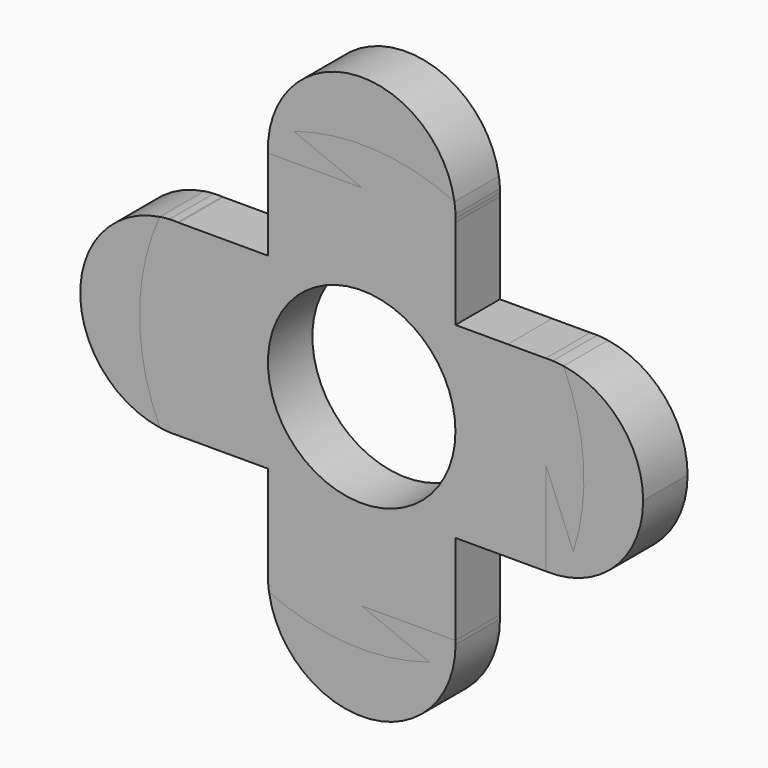
from build123d import *
from build123d import SkipClean  # not in build123d's __all__

# Parameters (mm, degrees)
F0_R     = 25.4
F1_DEPTH = 6.35
F2_R     = 10.715625
F3_DEPTH = 6.351
F5_DEPTH = 6.351
F7_DEPTH = 6.35


# Not quite as in the source:
# - ends of sketch curves that miss each other by under 0.0002 mm in the source are joined


with BuildPart() as f1:
    # F0 (on Front) → F1 (new body)
    with BuildSketch(Plane.XZ):
        Circle(F0_R)
    extrude(amount=F1_DEPTH)

    # F2 (on face) → F3 (cut, through all)
    with BuildSketch(Plane.XZ.offset(6.35)):
        Circle(F2_R)
    extrude(amount=-F3_DEPTH, mode=Mode.SUBTRACT)

    # F4 (on face) → F5 (cut, through all)
    with BuildSketch(Plane.XZ.offset(6.35)):
        Polygon((-16.6851454689, 10.715625), (-10.715625, 10.715625), (-10.715625, 16.6851454689), (-14.959796627, 14.959796627), align=None)
        with BuildLine():
            Line((-14.959796627, 14.959796627), (-10.715625, 16.6851454689))
            Line((-10.715625, 16.6851454689), (-10.715625, 21.0412820273))
            ThreePointArc((-10.715625, 21.0412820273), (-10.7231093189, 21.441908849), (-10.715625, 21.8425356707))
            Line((-10.715625, 21.8425356707), (-10.715625, 23.0290117213))
            ThreePointArc((-10.715625, 23.0290117213), (-11.3239040523, 22.7360769926), (-11.9241826151, 22.4270789217))
            Line((-11.9241826151, 22.4270789217), (-14.959796627, 14.959796627))
        make_face()
        with BuildLine():
            Line((-20.9014356742, 10.715625), (-16.6851454689, 10.715625))
            Line((-16.6851454689, 10.715625), (-14.959796627, 14.959796627))
            Line((-14.959796627, 14.959796627), (-22.4270789217, 11.9241826151))
            ThreePointArc((-22.4270789217, 11.9241826151), (-22.7360769926, 11.3239040523), (-23.0290117213, 10.715625))
            Line((-23.0290117213, 10.715625), (-21.9888344018, 10.715625))
            ThreePointArc((-21.9888344018, 10.715625), (-21.517375938, 10.7291661682), (-21.0457778798, 10.7219746652))
            ThreePointArc((-21.0457778798, 10.7219746652), (-20.9735960889, 10.7190427964), (-20.9014356742, 10.715625))
        make_face()
        Polygon((-10.715625, -16.6889140547), (-10.715625, -10.7183040998), (-16.6844990564, -10.7197962397), (-14.9584916016, -14.9648416016), align=None)
        Polygon((10.721975, 16.6873822364), (10.721975, 10.7183053524), (16.6882676196, 10.7197968469), (14.9635371125, 14.9635367777), align=None)
        with BuildLine():
            ThreePointArc((-10.715625, 21.8425356707), (-10.7231093189, 21.441908849), (-10.715625, 21.0412820273))
            Line((-10.715625, 21.0412820273), (-10.715625, 21.8425356707))
        make_face()
        with BuildLine():
            Line((-10.715625, 21.8425356707), (-10.715625, 21.0412820273))
            Line((-10.715625, 21.0412820273), (0, 21.0412820273))
            Line((0, 21.0412820273), (0.0045507281, 21.0431319981))
            Line((0.0045507281, 21.0431319981), (-7.7418402479, 24.1914015629))
            ThreePointArc((-7.7418402479, 24.1914015629), (-9.1859591102, 23.6807549547), (-10.596671596, 23.0839890635))
            ThreePointArc((-10.596671596, 23.0839890635), (-10.6742064582, 22.4649926613), (-10.715625, 21.8425356707))
        make_face()
        with BuildLine():
            Line((-22.4270789217, 11.9241826151), (-14.959796627, 14.959796627))
            Line((-14.959796627, 14.959796627), (-11.9241826151, 22.4270789217))
            ThreePointArc((-11.9241826151, 22.4270789217), (-17.9605122421, 17.9605122421), (-22.4270789217, 11.9241826151))
        make_face()
        with BuildLine():
            Line((-10.715625, -21.0430976268), (-10.715625, -16.6889140547))
            Line((-10.715625, -16.6889140547), (-14.9584916016, -14.9648416016))
            Line((-14.9584916016, -14.9648416016), (-11.9244537164, -22.4269347787))
            ThreePointArc((-11.9244537164, -22.4269347787), (-11.3240414708, -22.7360085496), (-10.715625, -23.0290117213))
            Line((-10.715625, -23.0290117213), (-10.715625, -21.8405802232))
            ThreePointArc((-10.715625, -21.8405802232), (-10.7230390601, -21.441838925), (-10.715625, -21.0430976268))
        make_face()
        with BuildLine():
            Line((-14.9584916016, -14.9648416016), (-16.6844990564, -10.7197962397))
            Line((-16.6844990564, -10.7197962397), (-21.0123347342, -10.7208781415))
            ThreePointArc((-21.0123347342, -10.7208781415), (-21.0263755955, -10.7214357653), (-21.0404171751, -10.721975))
            ThreePointArc((-21.0404171751, -10.721975), (-21.4565047306, -10.7296046859), (-21.8725751819, -10.7210931903))
            Line((-21.8725751819, -10.7210931903), (-23.0263322368, -10.7213816143))
            ThreePointArc((-23.0263322368, -10.7213816143), (-22.7327836194, -11.3305140622), (-22.4231246927, -11.9316167813))
            Line((-22.4231246927, -11.9316167813), (-14.9584916016, -14.9648416016))
        make_face()
        Polygon((16.6889139739, -10.7156253348), (10.721975, -10.7156253348), (10.721975, -16.6836133856), (14.9648415328, -14.9584918676), align=None)
        with BuildLine():
            Line((10.721975, 21.0412820273), (10.721975, 16.6873822364))
            Line((10.721975, 16.6873822364), (14.9635371125, 14.9635367777))
            Line((14.9635371125, 14.9635367777), (11.9318881389, 22.4229802979))
            ThreePointArc((11.9318881389, 22.4229802979), (11.3309445253, 22.7325690621), (10.721975, 23.0260559389))
            Line((10.721975, 23.0260559389), (10.721975, 21.8425356707))
            ThreePointArc((10.721975, 21.8425356707), (10.727588076, 21.6422572114), (10.7294593189, 21.441908849))
            ThreePointArc((10.7294593189, 21.441908849), (10.727588076, 21.2415604866), (10.721975, 21.0412820273))
        make_face()
        with BuildLine():
            Line((14.9635371125, 14.9635367777), (16.6882676196, 10.7197968469))
            Line((16.6882676196, 10.7197968469), (21.0404868941, 10.7208848444))
            ThreePointArc((21.0404868941, 10.7208848444), (21.4451864116, 10.7286236807), (21.8498897476, 10.7210871844))
            Line((21.8498897476, 10.7210871844), (23.0263323927, 10.7213812796))
            ThreePointArc((23.0263323927, 10.7213812796), (22.7327152374, 11.3306512582), (22.4229804989, 11.9318877612))
            Line((22.4229804989, 11.9318877612), (14.9635371125, 14.9635367777))
        make_face()
        with BuildLine():
            Line((-10.715625, 23.0290117213), (-10.715625, 21.8425356707))
            ThreePointArc((-10.715625, 21.8425356707), (-10.6742064582, 22.4649926613), (-10.596671596, 23.0839890635))
            ThreePointArc((-10.596671596, 23.0839890635), (-10.6561837529, 23.0565771055), (-10.715625, 23.0290117213))
        make_face()
        with BuildLine():
            Line((-11.9244537164, -22.4269347787), (-14.9584916016, -14.9648416016))
            Line((-14.9584916016, -14.9648416016), (-22.4231246927, -11.9316167813))
            ThreePointArc((-22.4231246927, -11.9316167813), (-17.9576435149, -17.9633805112), (-11.9244537164, -22.4269347787))
        make_face()
        with BuildLine():
            Line((14.9648415328, -14.9584918676), (10.721975, -16.6836133856))
            Line((10.721975, -16.6836133856), (10.721975, -21.0430976268))
            ThreePointArc((10.721975, -21.0430976268), (10.7275353849, -21.2424338153), (10.7293890601, -21.441838925))
            ThreePointArc((10.7293890601, -21.441838925), (10.7275353849, -21.6412440348), (10.721975, -21.8405802232))
            Line((10.721975, -21.8405802232), (10.721975, -23.0260559389))
            ThreePointArc((10.721975, -23.0260559389), (11.3308069807, -22.7326376201), (11.9316167956, -22.4231246851))
            Line((11.9316167956, -22.4231246851), (14.9648415328, -14.9584918676))
        make_face()
        with BuildLine():
            Line((21.0458457391, -10.7156253348), (16.6889139739, -10.7156253348))
            Line((16.6889139739, -10.7156253348), (14.9648415328, -14.9584918676))
            Line((14.9648415328, -14.9584918676), (22.4269345702, -11.9244541084))
            ThreePointArc((22.4269345702, -11.9244541084), (22.7360083683, -11.3240418348), (23.0290115655, -10.7156253348))
            Line((23.0290115655, -10.7156253348), (21.8498897476, -10.7156253348))
            ThreePointArc((21.8498897476, -10.7156253348), (21.4478677434, -10.7231621662), (21.0458457391, -10.7156253348))
        make_face()
        with BuildLine():
            Line((10.721975, -21.0430976268), (0, -21.0430976268))
            Line((0, -21.0430976268), (7.7450996927, -24.1903582187))
            ThreePointArc((7.7450996927, -24.1903582187), (9.1910155426, -23.678792902), (10.6034192636, -23.0808903624))
            ThreePointArc((10.6034192636, -23.0808903624), (10.6807217402, -22.462458185), (10.721975, -21.8405802232))
            Line((10.721975, -21.8405802232), (10.721975, -21.0430976268))
        make_face()
        with BuildLine():
            ThreePointArc((10.7293890601, -21.441838925), (10.7275353849, -21.2424338153), (10.721975, -21.0430976268))
            Line((10.721975, -21.0430976268), (10.721975, -21.8405802232))
            ThreePointArc((10.721975, -21.8405802232), (10.7275353849, -21.6412440348), (10.7293890601, -21.441838925))
        make_face()
        with BuildLine():
            ThreePointArc((-23.0806092952, 10.6040310525), (-22.536149575, 10.6737961307), (-21.9888344018, 10.715625))
            Line((-21.9888344018, 10.715625), (-23.0290117213, 10.715625))
            ThreePointArc((-23.0290117213, 10.715625), (-23.0548780277, 10.6598592451), (-23.0806092952, 10.6040310525))
        make_face()
        with BuildLine():
            Line((11.9318881389, 22.4229802979), (14.9635371125, 14.9635367777))
            Line((14.9635371125, 14.9635367777), (22.4229804989, 11.9318877612))
            ThreePointArc((22.4229804989, 11.9318877612), (17.9605123934, 17.9605120909), (11.9318881389, 22.4229802979))
        make_face()
        with BuildLine():
            ThreePointArc((10.6035074316, 23.0808498576), (10.6807078337, 22.4634116022), (10.721975, 21.8425356707))
            Line((10.721975, 21.8425356707), (10.721975, 23.0260559389))
            ThreePointArc((10.721975, 23.0260559389), (10.6627764128, 23.053528996), (10.6035074316, 23.0808498576))
        make_face()
        with BuildLine():
            ThreePointArc((-10.5965833938, -23.0840295525), (-10.674220495, -22.4640392514), (-10.715625, -21.8405802232))
            Line((-10.715625, -21.8405802232), (-10.715625, -23.0290117213))
            ThreePointArc((-10.715625, -23.0290117213), (-10.6561397042, -23.0565974637), (-10.5965833938, -23.0840295525))
        make_face()
        with BuildLine():
            Line((-23.0263322368, -10.7213816143), (-21.8725751819, -10.7210931903))
            ThreePointArc((-21.8725751819, -10.7210931903), (-22.4781957728, -10.6797622384), (-23.0805097356, -10.60424775))
            ThreePointArc((-23.0805097356, -10.60424775), (-23.0534953804, -10.6628490914), (-23.0263322368, -10.7213816143))
        make_face()
        with BuildLine():
            Line((22.4269345702, -11.9244541084), (14.9648415328, -14.9584918676))
            Line((14.9648415328, -14.9584918676), (11.9316167956, -22.4231246851))
            ThreePointArc((11.9316167956, -22.4231246851), (17.96338036, -17.9576436662), (22.4269345702, -11.9244541084))
        make_face()
        with BuildLine():
            Line((21.043166974, 0), (21.0458457391, -10.7156253348))
            Line((21.0458457391, -10.7156253348), (21.8498897476, -10.7156253348))
            ThreePointArc((21.8498897476, -10.7156253348), (22.4684041732, -10.6745013006), (23.083509992, -10.5977151524))
            ThreePointArc((23.083509992, -10.5977151524), (23.6805472866, -9.1864944461), (24.19140152, -7.7418403819))
            Line((24.19140152, -7.7418403819), (21.0440741561, 0.0022325353))
            Line((21.0440741561, 0.0022325353), (21.043166974, 0))
        make_face()
        with BuildLine():
            Line((21.8498897476, -10.7156253348), (21.0458457391, -10.7156253348))
            ThreePointArc((21.0458457391, -10.7156253348), (21.4478677434, -10.7231621662), (21.8498897476, -10.7156253348))
        make_face()
        with BuildLine():
            Line((10.721975, -23.0260559389), (10.721975, -21.8405802232))
            ThreePointArc((10.721975, -21.8405802232), (10.6807217402, -22.462458185), (10.6034192636, -23.0808903624))
            ThreePointArc((10.6034192636, -23.0808903624), (10.662732381, -23.0535493617), (10.721975, -23.0260559389))
        make_face()
        with BuildLine():
            Line((23.0263323927, 10.7213812796), (21.8498897476, 10.7210871844))
            ThreePointArc((21.8498897476, 10.7210871844), (22.467044649, 10.680093007), (23.0808104612, 10.603593186))
            ThreePointArc((23.0808104612, 10.603593186), (23.053646654, 10.6625220259), (23.0263323927, 10.7213812796))
        make_face()
        with BuildLine():
            ThreePointArc((23.083509992, -10.5977151524), (22.4684041732, -10.6745013006), (21.8498897476, -10.7156253348))
            Line((21.8498897476, -10.7156253348), (23.0290115655, -10.7156253348))
            ThreePointArc((23.0290115655, -10.7156253348), (23.056336153, -10.6567050818), (23.083509992, -10.5977151524))
        make_face()
    extrude(amount=-F5_DEPTH, mode=Mode.SUBTRACT)

    # F6 (on face) → F7 (join)
    with BuildSketch(Plane.XZ.offset(6.35)):
        with BuildLine():
            ThreePointArc((-23.0805097356, -10.60424775), (-25.3999999997, -0.0001192371), (-23.0806092952, 10.6040310525))
            ThreePointArc((-23.0806092952, 10.6040310525), (-32.1746450763, -0.0001510398), (-23.0805097356, -10.60424775))
        make_face()
        with BuildLine():
            ThreePointArc((-7.7418402479, 24.1914015629), (1.5348016289, 25.353587201), (10.6035074316, 23.0808498576))
            ThreePointArc((10.6035074316, 23.0808498576), (-1.0183277532, 32.1194416828), (-10.715625, 21.0412820273))
            Line((-10.715625, 21.0412820273), (0, 21.0412820273))
            Line((0, 21.0412820273), (0.0045507281, 21.0431319981))
            Line((0.0045507281, 21.0431319981), (-7.7418402479, 24.1914015629))
        make_face()
        with BuildLine():
            ThreePointArc((32.1737608344, 0.0027309248), (29.5891069493, 6.9859255227), (23.0808104612, 10.603593186))
            ThreePointArc((23.0808104612, 10.603593186), (25.353584354, 1.534848658), (24.19140152, -7.7418403819))
            Line((24.19140152, -7.7418403819), (21.0440741561, 0.0022325353))
            Line((21.0440741561, 0.0022325353), (21.043166974, 0))
            Line((21.043166974, 0), (21.0458457391, -10.7156253348))
            ThreePointArc((21.0458457391, -10.7156253348), (28.8887258109, -7.7224495792), (32.1737608344, 0.0027309248))
        make_face()
        with BuildLine():
            ThreePointArc((10.7293890601, -21.441838925), (10.7275353849, -21.2424338153), (10.721975, -21.0430976268))
            Line((10.721975, -21.0430976268), (0, -21.0430976268))
            Line((0, -21.0430976268), (7.7450996927, -24.1903582187))
            ThreePointArc((7.7450996927, -24.1903582187), (-1.5292908827, -25.3539201978), (-10.5965833938, -23.0840295525))
            ThreePointArc((-10.5965833938, -23.0840295525), (0.8267011217, -32.136392342), (10.7293890601, -21.441838925))
        make_face()
    with SkipClean():  # cleaning this boolean's faces spoils the solid; the shape is the same uncleaned
        extrude(amount=-F7_DEPTH)


solid = f1.part
